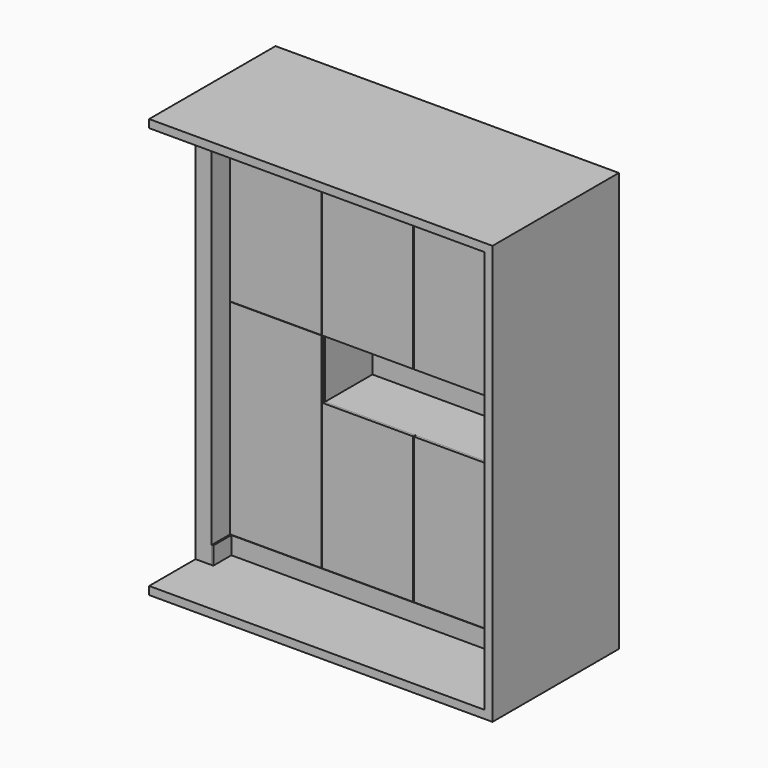
from build123d import *

# Parameters (mm, degrees)
F0_W      = 2080
F0_H      = 2600
F0_W_2    = 1710
F0_H_2    = 2500
F1_DEPTH  = 430
F2_W      = 100
F2_H      = 2600
F3_DEPTH  = 140
F4_W      = 2080
F4_H      = 50
F5_DEPTH  = 500
F6_W      = 930
F6_H      = 2600
F7_DEPTH  = 50
F8_W      = 2130
F8_H      = 2600
F9_DEPTH  = 50
F11_W     = 10
F11_H     = 110
F12_DEPTH = 570
F13_W     = 1700
F13_H     = 110
F14_DEPTH = 12
F15_W     = 1710
F15_H     = 100
F16_DEPTH = 16
F17_W     = 414
F17_H     = 2350
F18_DEPTH = 16
F22_DEPTH = 8
F24_DEPTH = 8
F23_W     = 414
F23_H     = 1050
F26_DEPTH = 16
F27_W     = 1116
F27_H     = 414
F28_DEPTH = 16
F29_W     = 1116
F29_H     = 414
F30_DEPTH = 16
F31_W     = 1700
F31_H     = 110
F32_DEPTH = 16
F34_W     = 546
F34_H     = 414
F35_DEPTH = 16
F36_W     = 566
F36_H     = 1014
F37_DEPTH = 16
F38_W     = 566
F38_H     = 1270
F39_DEPTH = 16
F38_H_2   = 904
F40_W     = 546
F40_H     = 16
F41_DEPTH = 414
F40_W_2   = 554
F42_W     = 28
F42_H     = 2390
F43_DEPTH = 28
F44_W     = 1116
F44_H     = 368
F45_DEPTH = 18
F47_W     = 546
F47_H     = 28
F48_DEPTH = 28
F47_W_2   = 526
F47_W_3   = 518
F49_W     = 28
F49_H     = 28
F50_DEPTH = 350
F51_W     = 28
F51_H     = 28
F52_DEPTH = 350


with BuildPart() as f1:
    # F0 (on Front) → F1 (new body)
    with BuildSketch(Plane.XZ):
        with Locations((940, 1250)):
            Rectangle(F0_W, F0_H)
        with Locations((855, 1250)):
            Rectangle(F0_W_2, F0_H_2, mode=Mode.SUBTRACT)
    extrude(amount=F1_DEPTH)

    # F2 (on face) → F3 (join)
    with BuildSketch(Plane.XZ.offset(430)):
        with Locations((-50, 1250)):
            Rectangle(F2_W, F2_H)
    extrude(amount=F3_DEPTH)

    # F4 (on face) → F5 (join)
    with BuildSketch(Plane.XZ.offset(430)):
        with Locations((940, 2525)):
            Rectangle(F4_W, F4_H)
        with Locations((940, -25)):
            Rectangle(F4_W, F4_H)
    extrude(amount=F5_DEPTH)

    # F6 (on face) → F7 (join)
    with BuildSketch(Plane.YZ.offset(1980)):
        with Locations((-465, 1250)):
            Rectangle(F6_W, F6_H)
    extrude(amount=F7_DEPTH)

    # F8 (on face) → F9 (join)
    with BuildSketch(Plane(origin=(0, 0, 0), x_dir=(-1, 0, 0), z_dir=(0, 1, 0))):
        with Locations((-965, 1250)):
            Rectangle(F8_W, F8_H)
    extrude(amount=F9_DEPTH)


with BuildPart() as f12:
    # F11 (on face) → F12 (new body, through all)
    with BuildSketch(Plane.XZ.offset(570)):
        with Locations((5, 55)):
            Rectangle(F11_W, F11_H)
    extrude(amount=-F12_DEPTH)

    # F13 (on face) → F14 (join)
    with BuildSketch(Plane.XZ):
        with Locations((860, 55)):
            Rectangle(F13_W, F13_H)
    extrude(amount=F14_DEPTH)


with BuildPart() as f16:
    # F15 (on face) → F16 (new body)
    with BuildSketch(Plane.XZ.offset(430)):
        with Locations((855, 2450)):
            Rectangle(F15_W, F15_H)
    extrude(amount=-F16_DEPTH)


with BuildPart() as f18:
    # F17 (on face) → F18 (new body)
    with BuildSketch(Plane.YZ):
        with Locations((-207, 1285)):
            Rectangle(F17_W, F17_H)
    extrude(amount=F18_DEPTH)


with BuildPart() as f22:
    # F21 (on line) → F22 (new body, symmetric)
    with BuildSketch(Plane.YZ.offset(570)):
        Polygon((-414, 2450), (-414, 0), (-14, 0), (-14, 112), (0, 112), (0, 2450), align=None)
    extrude(amount=F22_DEPTH, both=True)


with BuildPart() as f24:
    # F23 (on line) → F24 (new body, symmetric)
    with BuildSketch(Plane.YZ.offset(1140)):
        Polygon((-414, 1000), (-414, 0), (-14, 0), (-14, 112), (0, 112), (0, 1000), align=None)
    extrude(amount=F24_DEPTH, both=True)


with BuildPart() as f24b:
    # F23 (on line) → F24, piece 2 (new body, symmetric)
    with BuildSketch(Plane.YZ.offset(1140)):
        with Locations((-207, 1925)):
            Rectangle(F23_W, F23_H)
    extrude(amount=F24_DEPTH, both=True)


with BuildPart() as f26:
    # F25 (on face) → F26 (new body)
    with BuildSketch(Plane(origin=(1710, 0, 0), x_dir=(0, -1, 0), z_dir=(-1, 0, 0))):
        Polygon((414, 0), (414, 2450), (0, 2450), (0, 112), (14, 112), (14, 0), align=None)
    extrude(amount=F26_DEPTH)


with BuildPart() as f28:
    # F27 (on face) → F28 (new body)
    with BuildSketch(Plane(origin=(0, 0, 1400), x_dir=(1, 0, 0), z_dir=(0, 0, -1))):
        with Locations((1136, 207)):
            Rectangle(F27_W, F27_H)
    extrude(amount=F28_DEPTH)


with BuildPart() as f30:
    # F29 (on face) → F30 (new body)
    with BuildSketch(Plane.XY.offset(1000)):
        with Locations((1136, -207)):
            Rectangle(F29_W, F29_H)
    extrude(amount=F30_DEPTH)


with BuildPart() as f32:
    # F31 (on face) → F32 (new body)
    with BuildSketch(Plane.XZ.offset(414)):
        with Locations((860, 55)):
            Rectangle(F31_W, F31_H)
    extrude(amount=F32_DEPTH)


with BuildPart() as f35:
    # F34 (on offset) → F35 (new body)
    with BuildSketch(Plane.XY.offset(1391)):
        with Locations((289, -207)):
            Rectangle(F34_W, F34_H)
    extrude(amount=-F35_DEPTH)


with BuildPart() as f37:
    # F36 (on face) → F37 (new body)
    with BuildSketch(Plane.XZ.offset(414)):
        with Locations((285, 1891)):
            Rectangle(F36_W, F36_H)
    extrude(amount=F37_DEPTH)


with BuildPart() as f37b:
    # F36 (on face) → F37, piece 2 (new body)
    with BuildSketch(Plane.XZ.offset(414)):
        with Locations((855, 1891)):
            Rectangle(F36_W, F36_H)
    extrude(amount=F37_DEPTH)


with BuildPart() as f37c:
    # F36 (on face) → F37, piece 3 (new body)
    with BuildSketch(Plane.XZ.offset(414)):
        with Locations((1425, 1891)):
            Rectangle(F36_W, F36_H)
    extrude(amount=F37_DEPTH)


with BuildPart() as f39:
    # F38 (on face) → F39 (new body)
    with BuildSketch(Plane.XZ.offset(414)):
        with Locations((285, 747)):
            Rectangle(F38_W, F38_H)
    extrude(amount=F39_DEPTH)


with BuildPart() as f39b:
    # F38 (on face) → F39, piece 2 (new body)
    with BuildSketch(Plane.XZ.offset(414)):
        with Locations((855, 564)):
            Rectangle(F38_W, F38_H_2)
    extrude(amount=F39_DEPTH)


with BuildPart() as f39c:
    # F38 (on face) → F39, piece 3 (new body)
    with BuildSketch(Plane.XZ.offset(414)):
        with Locations((1425, 564)):
            Rectangle(F38_W, F38_H_2)
    extrude(amount=F39_DEPTH)


with BuildPart() as f41:
    # F40 (on face) → F41 (new body, through all)
    with BuildSketch(Plane.XZ.offset(414)):
        with Locations((289, 1849)):
            Rectangle(F40_W, F40_H)
    extrude(amount=-F41_DEPTH)


with BuildPart() as f41b:
    # F40 (on face) → F41, piece 2 (new body, through all)
    with BuildSketch(Plane.XZ.offset(414)):
        with Locations((855, 1849)):
            Rectangle(F40_W_2, F40_H)
    extrude(amount=-F41_DEPTH)


with BuildPart() as f41c:
    # F40 (on face) → F41, piece 3 (new body, through all)
    with BuildSketch(Plane.XZ.offset(414)):
        with Locations((1421, 1849)):
            Rectangle(F40_W, F40_H)
    extrude(amount=-F41_DEPTH)


with BuildPart() as f43:
    # F42 (on face) → F43 (new body)
    with BuildSketch(Plane.XZ):
        with Locations((592, 1305)):
            Rectangle(F42_W, F42_H)
    extrude(amount=F43_DEPTH)


with BuildPart() as f43b:
    # F42 (on face) → F43, piece 2 (new body)
    with BuildSketch(Plane.XZ):
        with Locations((1162, 1305)):
            Rectangle(F42_W, F42_H)
    extrude(amount=F43_DEPTH)


with BuildPart() as f45:
    # F44 (on face) → F45 (new body)
    with BuildSketch(Plane.XZ.offset(28)):
        with Locations((1136, 1200)):
            Rectangle(F44_W, F44_H)
    extrude(amount=F45_DEPTH)


with BuildPart() as f28_1:
    add(f28.part)

    # F46: cut F43, F43b
    add(f43.part, mode=Mode.SUBTRACT)
    add(f43b.part, mode=Mode.SUBTRACT)


with BuildPart() as f41b_1:
    add(f41b.part)

    # F46: cut F43, F43b
    add(f43.part, mode=Mode.SUBTRACT)
    add(f43b.part, mode=Mode.SUBTRACT)


with BuildPart() as f41c_1:
    add(f41c.part)

    # F46: cut F43, F43b
    add(f43.part, mode=Mode.SUBTRACT)
    add(f43b.part, mode=Mode.SUBTRACT)


with BuildPart() as f30_1:
    add(f30.part)

    # F46: cut F43, F43b
    add(f43.part, mode=Mode.SUBTRACT)
    add(f43b.part, mode=Mode.SUBTRACT)


with BuildPart() as f48:
    # F47 (on face) → F48 (new body)
    with BuildSketch(Plane.XZ):
        with Locations((289, 1827)):
            Rectangle(F47_W, F47_H)
    extrude(amount=F48_DEPTH)


with BuildPart() as f48b:
    # F47 (on face) → F48, piece 2 (new body)
    with BuildSketch(Plane.XZ):
        with Locations((869, 1827)):
            Rectangle(F47_W_2, F47_H)
    extrude(amount=F48_DEPTH)


with BuildPart() as f48c:
    # F47 (on face) → F48, piece 3 (new body)
    with BuildSketch(Plane.XZ):
        with Locations((1435, 1827)):
            Rectangle(F47_W_3, F47_H)
    extrude(amount=F48_DEPTH)


with BuildPart() as f48d:
    # F47 (on face) → F48, piece 4 (new body)
    with BuildSketch(Plane.XZ):
        with Locations((289, 1361)):
            Rectangle(F47_W, F47_H)
    extrude(amount=F48_DEPTH)


with BuildPart() as f48e:
    # F47 (on face) → F48, piece 5 (new body)
    with BuildSketch(Plane.XZ):
        with Locations((869, 986)):
            Rectangle(F47_W_2, F47_H)
    extrude(amount=F48_DEPTH)


with BuildPart() as f48f:
    # F47 (on face) → F48, piece 6 (new body)
    with BuildSketch(Plane.XZ):
        with Locations((1435, 986)):
            Rectangle(F47_W_3, F47_H)
    extrude(amount=F48_DEPTH)


with BuildPart() as f50:
    # F49 (on face) → F50 (new body)
    with BuildSketch(Plane.XZ.offset(28)):
        with Locations((30, 1827)):
            Rectangle(F49_W, F49_H)
    extrude(amount=F50_DEPTH)


with BuildPart() as f50b:
    # F49 (on face) → F50, piece 2 (new body)
    with BuildSketch(Plane.XZ.offset(28)):
        with Locations((548, 1827)):
            Rectangle(F49_W, F49_H)
    extrude(amount=F50_DEPTH)


with BuildPart() as f50c:
    # F49 (on face) → F50, piece 3 (new body)
    with BuildSketch(Plane.XZ.offset(28)):
        with Locations((592, 1827)):
            Rectangle(F49_W, F49_H)
    extrude(amount=F50_DEPTH)


with BuildPart() as f50d:
    # F49 (on face) → F50, piece 4 (new body)
    with BuildSketch(Plane.XZ.offset(28)):
        with Locations((1118, 1827)):
            Rectangle(F49_W, F49_H)
    extrude(amount=F50_DEPTH)


with BuildPart() as f50e:
    # F49 (on face) → F50, piece 5 (new body)
    with BuildSketch(Plane.XZ.offset(28)):
        with Locations((1162, 1827)):
            Rectangle(F49_W, F49_H)
    extrude(amount=F50_DEPTH)


with BuildPart() as f50f:
    # F49 (on face) → F50, piece 6 (new body)
    with BuildSketch(Plane.XZ.offset(28)):
        with Locations((1680, 1827)):
            Rectangle(F49_W, F49_H)
    extrude(amount=F50_DEPTH)


with BuildPart() as f50g:
    # F49 (on face) → F50, piece 7 (new body)
    with BuildSketch(Plane.XZ.offset(28)):
        with Locations((30, 1361)):
            Rectangle(F49_W, F49_H)
    extrude(amount=F50_DEPTH)


with BuildPart() as f50h:
    # F49 (on face) → F50, piece 8 (new body)
    with BuildSketch(Plane.XZ.offset(28)):
        with Locations((548, 1361)):
            Rectangle(F49_W, F49_H)
    extrude(amount=F50_DEPTH)


with BuildPart() as f50i:
    # F49 (on face) → F50, piece 9 (new body)
    with BuildSketch(Plane.XZ.offset(28)):
        with Locations((592, 986)):
            Rectangle(F49_W, F49_H)
    extrude(amount=F50_DEPTH)


with BuildPart() as f50j:
    # F49 (on face) → F50, piece 10 (new body)
    with BuildSketch(Plane.XZ.offset(28)):
        with Locations((1118, 986)):
            Rectangle(F49_W, F49_H)
    extrude(amount=F50_DEPTH)


with BuildPart() as f50k:
    # F49 (on face) → F50, piece 11 (new body)
    with BuildSketch(Plane.XZ.offset(28)):
        with Locations((1680, 986)):
            Rectangle(F49_W, F49_H)
    extrude(amount=F50_DEPTH)


with BuildPart() as f52:
    # F51 (on face) → F52 (new body)
    with BuildSketch(Plane.XZ.offset(12)):
        with Locations((592, 14)):
            Rectangle(F51_W, F51_H)
    extrude(amount=F52_DEPTH)


with BuildPart() as f52b:
    # F51 (on face) → F52, piece 2 (new body)
    with BuildSketch(Plane.XZ.offset(12)):
        with Locations((1162, 14)):
            Rectangle(F51_W, F51_H)
    extrude(amount=F52_DEPTH)


solid = Compound([f1.part, f12.part, f16.part, f18.part, f22.part, f24.part, f24b.part, f26.part, f32.part, f35.part, f37.part, f37b.part, f37c.part, f39.part, f39b.part, f39c.part, f41.part, f43.part, f43b.part, f45.part, f28_1.part, f41b_1.part, f41c_1.part, f30_1.part, f48.part, f48b.part, f48c.part, f48d.part, f48e.part, f48f.part, f50.part, f50b.part, f50c.part, f50d.part, f50e.part, f50f.part, f50g.part, f50h.part, f50i.part, f50j.part, f50k.part, f52.part, f52b.part])
